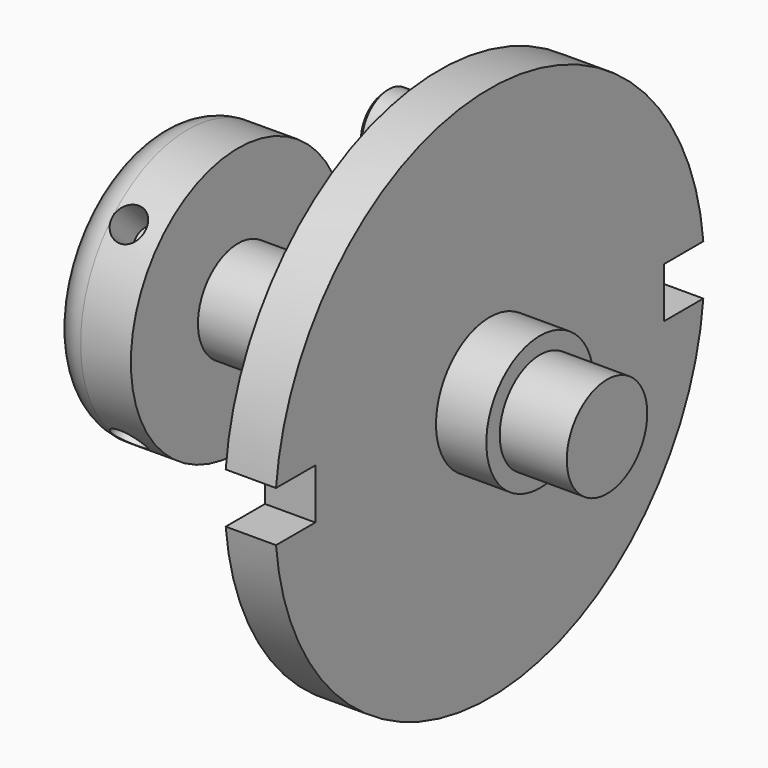
from build123d import *

# Parameters (mm, degrees)
F3_DEPTH        = 25.4
F4_R            = 12.7
F5_DEPTH        = 20.828
F6_SIZE         = 1.5875
F9_COPIES_COUNT = 4


# Not quite as in the source:
# - a pattern or mirror of a feature is missing from the dataset's text; its kind, count and spacing are read off the source's solid


with BuildPart() as f1:
    # F0 (on Top) → F1 (revolve)
    with BuildSketch(Plane.XY):
        with BuildLine():
            Line((-85.725, 38.1), (-85.725, 0))
            Line((-85.725, 0), (85.725, 0))
            Line((85.725, 0), (85.725, 19.05))
            Line((85.725, 19.05), (60.325, 19.05))
            Line((60.325, 19.05), (60.325, 25.4))
            Line((60.325, 25.4), (41.275, 25.4))
            Line((41.275, 25.4), (41.275, 101.6))
            Line((41.275, 101.6), (22.225, 101.6))
            Line((22.225, 101.6), (22.225, 19.05))
            Line((22.225, 19.05), (-53.975, 19.05))
            Line((-53.975, 19.05), (-53.975, 50.8))
            Line((-53.975, 50.8), (-73.025, 50.8))
            ThreePointArc((-73.025, 50.8), (-82.0052561211, 47.0802561211), (-85.725, 38.1))
        make_face()
    revolve(axis=Axis((0, 0, 0), (1, 0, 0)))

    # F2 (on face) → F3 (cut)
    with BuildSketch(Plane(origin=(22.225, 0, 0), x_dir=(0, -1, 0), z_dir=(-1, 0, 0))):
        with BuildLine():
            ThreePointArc((-101.1525302452, -9.525), (-101.6, 0), (-101.1525302452, 9.525))
            Line((-101.1525302452, 9.525), (-107.95, 9.525))
            Line((-107.95, 9.525), (-107.95, -9.525))
            Line((-107.95, -9.525), (-101.1525302452, -9.525))
        make_face()
        with BuildLine():
            ThreePointArc((101.1525302452, 9.525), (101.4880709071, 4.7677524627), (101.6, 0))
            ThreePointArc((101.6, 0), (101.4880709071, -4.7677524627), (101.1525302452, -9.525))
            Line((101.1525302452, -9.525), (107.95, -9.525))
            Line((107.95, -9.525), (107.95, 9.525))
            Line((107.95, 9.525), (101.1525302452, 9.525))
        make_face()
        with BuildLine():
            ThreePointArc((101.1525302452, -9.525), (101.4880709071, -4.7677524627), (101.6, 0))
            ThreePointArc((101.6, 0), (101.4880709071, 4.7677524627), (101.1525302452, 9.525))
            Line((101.1525302452, 9.525), (82.55, 9.525))
            Line((82.55, 9.525), (82.55, -9.525))
            Line((82.55, -9.525), (101.1525302452, -9.525))
        make_face()
        with BuildLine():
            Line((-82.55, 9.525), (-101.1525302452, 9.525))
            ThreePointArc((-101.1525302452, 9.525), (-101.6, 0), (-101.1525302452, -9.525))
            Line((-101.1525302452, -9.525), (-82.55, -9.525))
            Line((-82.55, -9.525), (-82.55, 9.525))
        make_face()
    extrude(amount=-F3_DEPTH, mode=Mode.SUBTRACT)

    # F4 (on face) → F5 (join)
    with BuildSketch(Plane(origin=(22.225, 0, 0), x_dir=(0, -1, 0), z_dir=(-1, 0, 0))):
        with Locations((0, 76.2)):
            Circle(F4_R)
        with Locations((0, -76.2)):
            Circle(F4_R)
    extrude(amount=F5_DEPTH)

    # F6
    f6_edges = [f1.edges().sort_by_distance(p)[0] for p in [
        (1.397, 12.7, 76.2),
        (1.397, 12.7, -76.2),
    ]]
    chamfer(f6_edges, length=F6_SIZE)

    # F8 (on offset) → F9 (revolve, cut)
    with BuildSketch(Plane.YZ.offset(-66.675)):
        Polygon((24.6957043329, -24.6957043329), (35.9210244843, -35.9210244843), (39.5131269327, -39.5131269327), (44.0032549932, -35.0229988722), (29.1858323935, -20.2055762724), align=None)
    f9 = revolve(axis=Axis((-66.675, 30.3083644086, -30.3083644086), (0, -0.7071067812, 0.7071067812)), mode=Mode.SUBTRACT)

    # F9_copies: F9 ×4 about axis
    f9_copies_axis = Axis((0, 0, 0), (1, 0, 0))
    for i in range(1, F9_COPIES_COUNT):
        add(f9.rotate(f9_copies_axis, i * 360 / F9_COPIES_COUNT), mode=Mode.SUBTRACT)


solid = f1.part
